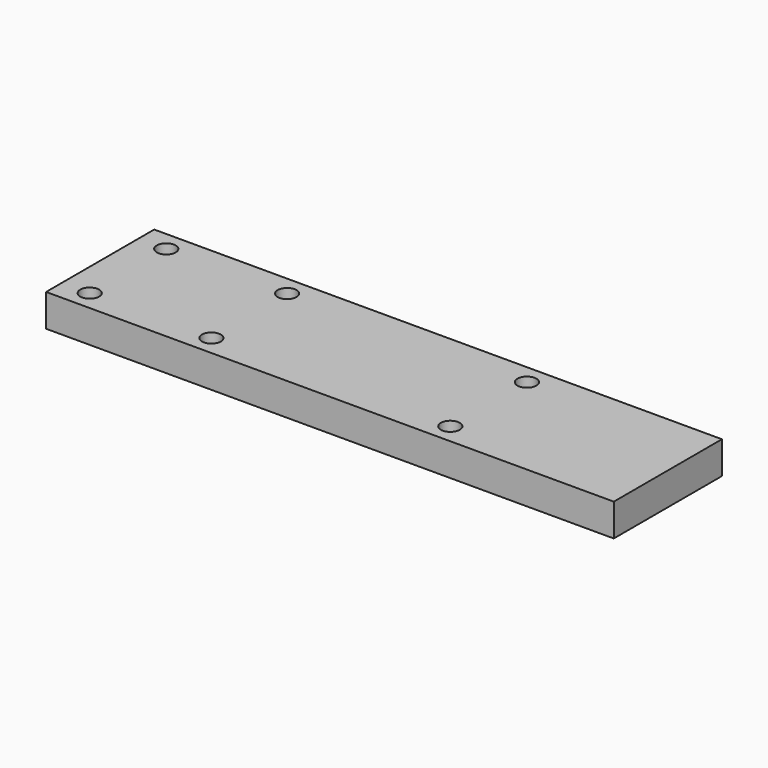
from build123d import *

# Parameters (mm, degrees)
F0_W     = 210
F0_H     = 50
F1_DEPTH = 12
F2_R     = 3.5
F3_DEPTH = 25
F4_R     = 3.5
F5_DEPTH = 25


# Not quite as in the source:
# - a feature names something its author has since deleted; it is built from what else it names


with BuildPart() as f1:
    # F0 (on Top) → F1 (new body)
    with BuildSketch(Plane.XY):
        with Locations((80.6913864613, -4.2518138885)):
            Rectangle(F0_W, F0_H)
    extrude(amount=F1_DEPTH)

    # F2 (on face) → F3 (cut)
    with BuildSketch(Plane.XY.offset(12)):
        with Locations((119.3913864613, 13.4481861115)):
            Circle(F2_R)
        with Locations((119.3913864613, -21.9518138885)):
            Circle(F2_R)
        with Locations((30.9913864613, -21.9518138885)):
            Circle(F2_R)
        with Locations((-14.0086135387, 13.4481861115)):
            Circle(F2_R)
        with Locations((-14.0086135387, -21.9518138885)):
            Circle(F2_R)
    extrude(amount=-F3_DEPTH, mode=Mode.SUBTRACT)

    # F4 (on face) → F5 (cut)
    with BuildSketch(Plane.XY.offset(12)):
        with Locations((30.6913864613, 13.4481861115)):
            Circle(F4_R)
    extrude(amount=-F5_DEPTH, mode=Mode.SUBTRACT)


solid = f1.part
